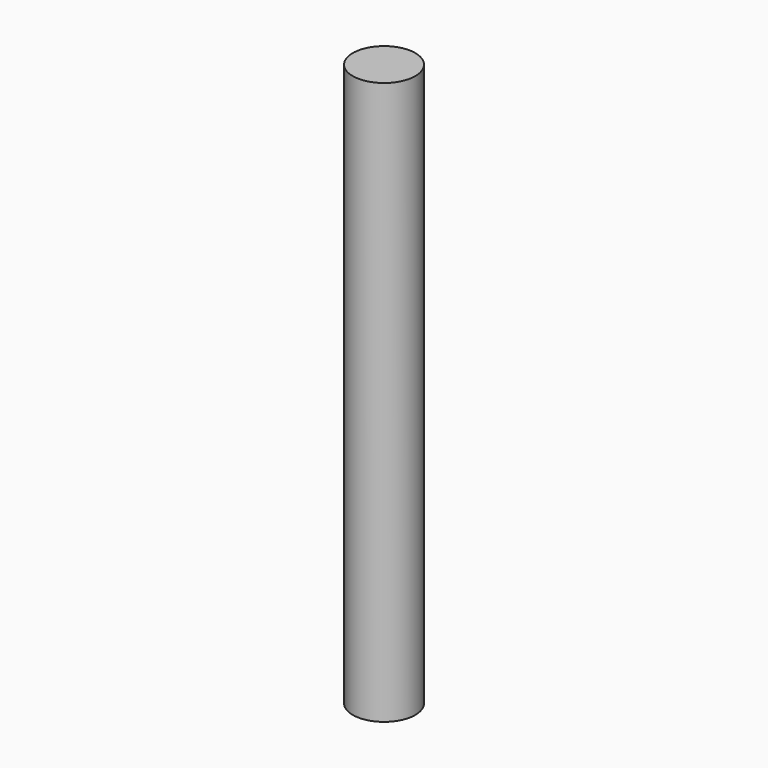
from build123d import *

# Parameters (mm, degrees)
F2_R     = 5
F3_DEPTH = 90


# Not quite as in the source:
# - the program builds the solid bodies; features that only make, move or delete a surface that nothing else refers to are left out


with BuildPart() as f3:
    # F2 (on Top) → F3 (new body)
    with BuildSketch(Plane.XY):
        Circle(F2_R)
    extrude(amount=F3_DEPTH)


solid = f3.part
